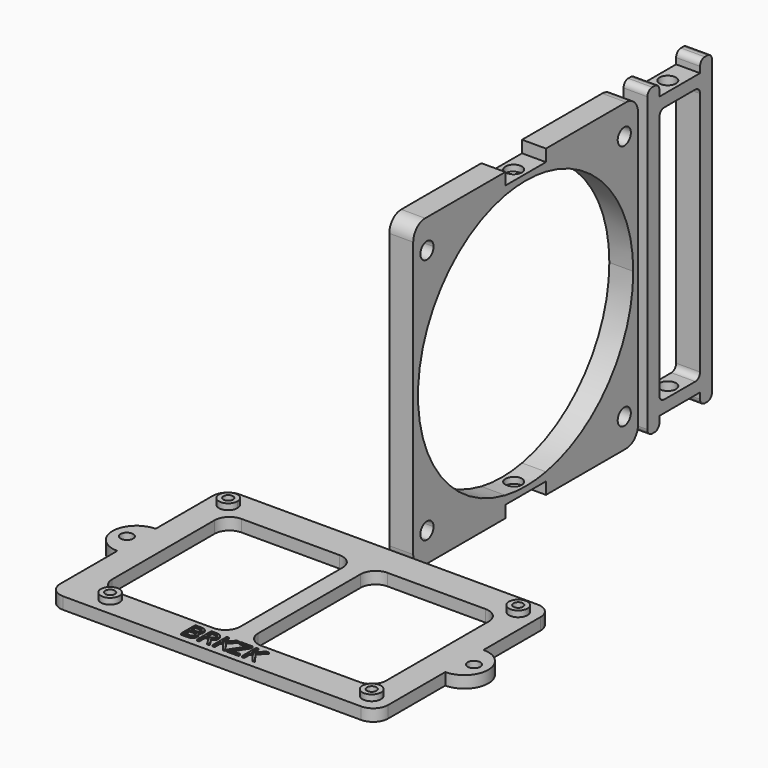
from build123d import *

# Parameters (mm, degrees)
F3_R      = 3.1
F3_W      = 42.85
F3_H      = 52.8
F3_R_2    = 2.1
F3_R_3    = 1.6
F3_W_2    = 0.69140625
F3_H_2    = 0.75
F4_DEPTH  = 4
F5_DEPTH  = 2
F6_DEPTH  = 0.4
F7_R      = 5
F8_R      = 5
F10_R     = 2.75
F10_W     = 38.5
F10_H     = 4
F11_DEPTH = 8
F13_D     = 5.5
F14_R     = 5
F15_W     = 17
F15_H     = 4
F16_DEPTH = 8
F18_D     = 5.5
F19_R     = 2


# Not quite as in the source:
# - a feature names something its author has since deleted; it is built from what else it names


with BuildPart() as f4:
    # F3 (on Top) → F4 (new body)
    with BuildSketch(Plane.XY):
        Polygon((54.85, 36.9), (-54.85, 36.9), (-54.85, 8), (-54.85, -8), (-54.85, -36.9), (-13.0384114583, -36.9), (54.85, -36.9), (54.85, -8), (54.85, 8), align=None)
        with BuildLine():
            Line((-51.85, -33.9), (-51.85, 33.9))
            Line((-51.85, 33.9), (-48.55, 33.9))
            Line((-48.55, 33.9), (51.85, 33.9))
            Line((51.85, 33.9), (51.85, -33.9))
            Line((51.85, -33.9), (11.9448348007, -33.9))
            Line((11.9448348007, -33.9), (12.498046875, -34.65))
            Line((12.498046875, -34.65), (11.6842447917, -34.65))
            Line((11.6842447917, -34.65), (11.1207294487, -33.9))
            Line((11.1207294487, -33.9), (8.892578125, -33.9))
            Line((8.892578125, -33.9), (8.892578125, -34.65))
            Line((8.892578125, -34.65), (8.201171875, -34.65))
            Line((8.201171875, -34.65), (8.201171875, -33.9))
            Line((8.201171875, -33.9), (3.8844248565, -33.9))
            Line((3.8844248565, -33.9), (3.802734375, -34.0236979167))
            Line((3.802734375, -34.0236979167), (7.0501302083, -34.0236979167))
            Line((7.0501302083, -34.0236979167), (7.0501302083, -34.65))
            Line((7.0501302083, -34.65), (2.9602864583, -34.65))
            Line((2.9602864583, -34.65), (2.9602864583, -34.1083333333))
            Line((2.9602864583, -34.1083333333), (3.0977581137, -33.9))
            Line((3.0977581137, -33.9), (2.0737410507, -33.9))
            Line((2.0737410507, -33.9), (2.626953125, -34.65))
            Line((2.626953125, -34.65), (1.8131510417, -34.65))
            Line((1.8131510417, -34.65), (1.2496356987, -33.9))
            Line((1.2496356987, -33.9), (-0.978515625, -33.9))
            Line((-0.978515625, -33.9), (-0.978515625, -34.65))
            Line((-0.978515625, -34.65), (-1.669921875, -34.65))
            Line((-1.669921875, -34.65), (-1.669921875, -33.9))
            Line((-1.669921875, -33.9), (-3.0829182269, -33.9))
            Line((-3.0829182269, -33.9), (-2.6295572917, -34.65))
            Line((-2.6295572917, -34.65), (-3.447265625, -34.65))
            Line((-3.447265625, -34.65), (-3.8838445724, -33.9))
            Line((-3.8838445724, -33.9), (-6.1295572917, -33.9))
            Line((-6.1295572917, -33.9), (-6.1295572917, -34.65))
            Line((-6.1295572917, -34.65), (-6.8209635417, -34.65))
            Line((-6.8209635417, -34.65), (-6.8209635417, -33.9))
            Line((-6.8209635417, -33.9), (-8.3611343756, -33.9))
            add(Edge.make_bspline(
                [(-8.3611343756, -33.9), (-8.4747116287, -34.0669277583), (-8.6373697917, -34.2020833333)],
                knots=[0.6982573208, 0.6982573208, 0.6982573208, 1, 1, 1], degree=2))
            add(Edge.make_bspline(
                [(-8.6373697917, -34.2020833333), (-9.1764322917, -34.65), (-10.1451822917, -34.65)],
                knots=[0, 0, 0, 1, 1, 1], degree=2))
            Line((-10.1451822917, -34.65), (-12.220703125, -34.65))
            Line((-12.220703125, -34.65), (-12.220703125, -33.9))
            Line((-12.220703125, -33.9), (-51.85, -33.9))
        make_face(mode=Mode.SUBTRACT)
        with BuildLine():
            Line((-48.55, 33.9), (-51.85, 33.9))
            Line((-51.85, 33.9), (-51.85, -33.9))
            Line((-51.85, -33.9), (-12.220703125, -33.9))
            Line((-12.220703125, -33.9), (-12.220703125, -28.70078125))
            Line((-12.220703125, -28.70078125), (-10.5397135417, -28.70078125))
            add(Edge.make_bspline(
                [(-10.5397135417, -28.70078125), (-9.3561197917, -28.70078125), (-8.8268229167, -29.0549479167)],
                knots=[0, 0, 0, 1, 1, 1], degree=2))
            add(Edge.make_bspline(
                [(-8.8268229167, -29.0549479167), (-8.2975260417, -29.4091145833), (-8.2975260417, -30.1734375)],
                knots=[0, 0, 0, 1, 1, 1], degree=2))
            add(Edge.make_bspline(
                [(-8.2975260417, -30.1734375), (-8.2975260417, -30.7033854167), (-8.5924479167, -31.0471354167)],
                knots=[0, 0, 0, 1, 1, 1], degree=2))
            add(Edge.make_bspline(
                [(-8.5924479167, -31.0471354167), (-8.8873697917, -31.3908854167), (-9.4537760417, -31.4924479167)],
                knots=[0, 0, 0, 1, 1, 1], degree=2))
            Line((-9.4537760417, -31.4924479167), (-9.4537760417, -31.5328125))
            add(Edge.make_bspline(
                [(-9.4537760417, -31.5328125), (-8.0983072917, -31.7645833333), (-8.0983072917, -32.9572916667)],
                knots=[0, 0, 0, 1, 1, 1], degree=2))
            add(Edge.make_bspline(
                [(-8.0983072917, -32.9572916667), (-8.0983072917, -33.5137154692), (-8.3611343756, -33.9)],
                knots=[0, 0, 0, 0.6982573208, 0.6982573208, 0.6982573208], degree=2))
            Line((-8.3611343756, -33.9), (-6.8209635417, -33.9))
            Line((-6.8209635417, -33.9), (-6.8209635417, -28.70078125))
            Line((-6.8209635417, -28.70078125), (-5.189453125, -28.70078125))
            add(Edge.make_bspline(
                [(-5.189453125, -28.70078125), (-4.0944010417, -28.70078125), (-3.5716145833, -29.1200520833)],
                knots=[0, 0, 0, 1, 1, 1], degree=2))
            add(Edge.make_bspline(
                [(-3.5716145833, -29.1200520833), (-3.048828125, -29.5393229167), (-3.048828125, -30.3817708333)],
                knots=[0, 0, 0, 1, 1, 1], degree=2))
            add(Edge.make_bspline(
                [(-3.048828125, -30.3817708333), (-3.048828125, -31.5614583333), (-4.2454427083, -31.9768229167)],
                knots=[0, 0, 0, 1, 1, 1], degree=2))
            Line((-4.2454427083, -31.9768229167), (-3.0829182269, -33.9))
            Line((-3.0829182269, -33.9), (-1.669921875, -33.9))
            Line((-1.669921875, -33.9), (-1.669921875, -28.70078125))
            Line((-1.669921875, -28.70078125), (-0.978515625, -28.70078125))
            Line((-0.978515625, -28.70078125), (-0.978515625, -31.6513020833))
            Line((-0.978515625, -31.6513020833), (1.7194010417, -28.70078125))
            Line((1.7194010417, -28.70078125), (2.537109375, -28.70078125))
            Line((2.537109375, -28.70078125), (0.1451822917, -31.2854166667))
            Line((0.1451822917, -31.2854166667), (2.0737410507, -33.9))
            Line((2.0737410507, -33.9), (3.0977581137, -33.9))
            Line((3.0977581137, -33.9), (6.1178385417, -29.3231770833))
            Line((6.1178385417, -29.3231770833), (3.0579427083, -29.3231770833))
            Line((3.0579427083, -29.3231770833), (3.0579427083, -28.70078125))
            Line((3.0579427083, -28.70078125), (6.9602864583, -28.70078125))
            Line((6.9602864583, -28.70078125), (6.9602864583, -29.2424479167))
            Line((6.9602864583, -29.2424479167), (3.8844248565, -33.9))
            Line((3.8844248565, -33.9), (8.201171875, -33.9))
            Line((8.201171875, -33.9), (8.201171875, -28.70078125))
            Line((8.201171875, -28.70078125), (8.892578125, -28.70078125))
            Line((8.892578125, -28.70078125), (8.892578125, -31.6513020833))
            Line((8.892578125, -31.6513020833), (11.5904947917, -28.70078125))
            Line((11.5904947917, -28.70078125), (12.408203125, -28.70078125))
            Line((12.408203125, -28.70078125), (10.0162760417, -31.2854166667))
            Line((10.0162760417, -31.2854166667), (11.9448348007, -33.9))
            Line((11.9448348007, -33.9), (51.85, -33.9))
            Line((51.85, -33.9), (51.85, 33.9))
            Line((51.85, 33.9), (-48.55, 33.9))
        make_face()
        with Locations((-39.25, -30.5)):
            Circle(F3_R, mode=Mode.SUBTRACT)
        with Locations((48.25, -30.5)):
            Circle(F3_R, mode=Mode.SUBTRACT)
        Polygon((-45.85, -26.4), (-45.85, 26.4), (-3, 26.4), (-3, -26.4), (-13.0384114583, -26.4), align=None, mode=Mode.SUBTRACT)
        with BuildLine():
            ThreePointArc((-45.45, 30.5), (-50.7420310217, 28.3079689783), (-48.55, 33.6))
            ThreePointArc((-48.55, 33.6), (-46.3579689783, 32.6920310217), (-45.45, 30.5))
        make_face(mode=Mode.SUBTRACT)
        with Locations((24.425, 0)):
            Rectangle(F3_W, F3_H, mode=Mode.SUBTRACT)
        with Locations((48.45, 30.5)):
            Circle(F3_R, mode=Mode.SUBTRACT)
        with BuildLine():
            ThreePointArc((54.85, -8), (62.85, 0), (54.85, 8))
            Line((54.85, 8), (54.85, -8))
        make_face()
        with Locations((58.05, 0)):
            Circle(F3_R_2, mode=Mode.SUBTRACT)
        with BuildLine():
            Line((-54.85, -8), (-54.85, 8))
            ThreePointArc((-54.85, 8), (-62.85, 0), (-54.85, -8))
        make_face()
        with Locations((-58.05, 0)):
            Circle(F3_R_2, mode=Mode.SUBTRACT)
        with BuildLine():
            ThreePointArc((-45.45, 30.5), (-46.3579689783, 32.6920310217), (-48.55, 33.6))
            ThreePointArc((-48.55, 33.6), (-50.7420310217, 28.3079689783), (-45.45, 30.5))
        make_face()
        with BuildLine():
            ThreePointArc((-46.95, 30.5), (-49.6813708499, 29.3686291501), (-48.55, 32.1))
            ThreePointArc((-48.55, 32.1), (-47.4186291501, 31.6313708499), (-46.95, 30.5))
        make_face(mode=Mode.SUBTRACT)
        with Locations((-39.25, -30.5)):
            Circle(F3_R)
        with Locations((-39.25, -30.5)):
            Circle(F3_R_3, mode=Mode.SUBTRACT)
        with Locations((48.25, -30.5)):
            Circle(F3_R)
        with Locations((48.25, -30.5)):
            Circle(F3_R_3, mode=Mode.SUBTRACT)
        with Locations((48.45, 30.5)):
            Circle(F3_R)
        with Locations((48.45, 30.5)):
            Circle(F3_R_3, mode=Mode.SUBTRACT)
        with BuildLine():
            Line((-6.8209635417, -28.70078125), (-6.8209635417, -33.9))
            Line((-6.8209635417, -33.9), (-6.1295572917, -33.9))
            Line((-6.1295572917, -33.9), (-6.1295572917, -32.1760416667))
            Line((-6.1295572917, -32.1760416667), (-4.8873697917, -32.1760416667))
            Line((-4.8873697917, -32.1760416667), (-3.8838445724, -33.9))
            Line((-3.8838445724, -33.9), (-3.0829182269, -33.9))
            Line((-3.0829182269, -33.9), (-4.2454427083, -31.9768229167))
            add(Edge.make_bspline(
                [(-3.048828125, -30.3817708333), (-3.048828125, -31.5614583333), (-4.2454427083, -31.9768229167)],
                knots=[0, 0, 0, 1, 1, 1], degree=2))
            add(Edge.make_bspline(
                [(-3.5716145833, -29.1200520833), (-3.048828125, -29.5393229167), (-3.048828125, -30.3817708333)],
                knots=[0, 0, 0, 1, 1, 1], degree=2))
            add(Edge.make_bspline(
                [(-5.189453125, -28.70078125), (-4.0944010417, -28.70078125), (-3.5716145833, -29.1200520833)],
                knots=[0, 0, 0, 1, 1, 1], degree=2))
            Line((-5.189453125, -28.70078125), (-6.8209635417, -28.70078125))
        make_face()
        with BuildLine():
            Line((-5.1803385417, -31.5822916667), (-6.1295572917, -31.5822916667))
            Line((-6.1295572917, -31.5822916667), (-6.1295572917, -29.3075520833))
            Line((-6.1295572917, -29.3075520833), (-5.2298177083, -29.3075520833))
            add(Edge.make_bspline(
                [(-4.1126302083, -29.56796875), (-4.4602864583, -29.3075520833), (-5.2298177083, -29.3075520833)],
                knots=[0, 0, 0, 1, 1, 1], degree=2))
            add(Edge.make_bspline(
                [(-3.7649739583, -30.4182291667), (-3.7649739583, -29.8283854167), (-4.1126302083, -29.56796875)],
                knots=[0, 0, 0, 1, 1, 1], degree=2))
            add(Edge.make_bspline(
                [(-4.1067708333, -31.2912760417), (-3.7649739583, -31.0002604167), (-3.7649739583, -30.4182291667)],
                knots=[0, 0, 0, 1, 1, 1], degree=2))
            add(Edge.make_bspline(
                [(-5.1803385417, -31.5822916667), (-4.4485677083, -31.5822916667), (-4.1067708333, -31.2912760417)],
                knots=[0, 0, 0, 1, 1, 1], degree=2))
        make_face(mode=Mode.SUBTRACT)
        with BuildLine():
            Line((-12.220703125, -28.70078125), (-12.220703125, -33.9))
            Line((-12.220703125, -33.9), (-11.529296875, -33.9))
            Line((-11.529296875, -33.9), (-11.529296875, -31.83359375))
            Line((-11.529296875, -31.83359375), (-10.3444010417, -31.83359375))
            add(Edge.make_bspline(
                [(-9.2115885417, -32.0940104167), (-9.583984375, -31.83359375), (-10.3444010417, -31.83359375)],
                knots=[0, 0, 0, 1, 1, 1], degree=2))
            add(Edge.make_bspline(
                [(-8.8391927083, -32.9078125), (-8.8391927083, -32.3544270833), (-9.2115885417, -32.0940104167)],
                knots=[0, 0, 0, 1, 1, 1], degree=2))
            add(Edge.make_bspline(
                [(-9.203125, -33.7815104167), (-8.8391927083, -33.5028645833), (-8.8391927083, -32.9078125)],
                knots=[0, 0, 0, 1, 1, 1], degree=2))
            add(Edge.make_bspline(
                [(-9.4000038836, -33.9), (-9.2911480413, -33.8489055181), (-9.203125, -33.7815104167)],
                knots=[0.7581334679, 0.7581334679, 0.7581334679, 1, 1, 1], degree=2))
            Line((-9.4000038836, -33.9), (-8.3611343756, -33.9))
            add(Edge.make_bspline(
                [(-8.0983072917, -32.9572916667), (-8.0983072917, -33.5137154692), (-8.3611343756, -33.9)],
                knots=[0, 0, 0, 0.6982573208, 0.6982573208, 0.6982573208], degree=2))
            add(Edge.make_bspline(
                [(-9.4537760417, -31.5328125), (-8.0983072917, -31.7645833333), (-8.0983072917, -32.9572916667)],
                knots=[0, 0, 0, 1, 1, 1], degree=2))
            Line((-9.4537760417, -31.5328125), (-9.4537760417, -31.4924479167))
            add(Edge.make_bspline(
                [(-8.5924479167, -31.0471354167), (-8.8873697917, -31.3908854167), (-9.4537760417, -31.4924479167)],
                knots=[0, 0, 0, 1, 1, 1], degree=2))
            add(Edge.make_bspline(
                [(-8.2975260417, -30.1734375), (-8.2975260417, -30.7033854167), (-8.5924479167, -31.0471354167)],
                knots=[0, 0, 0, 1, 1, 1], degree=2))
            add(Edge.make_bspline(
                [(-8.8268229167, -29.0549479167), (-8.2975260417, -29.4091145833), (-8.2975260417, -30.1734375)],
                knots=[0, 0, 0, 1, 1, 1], degree=2))
            add(Edge.make_bspline(
                [(-10.5397135417, -28.70078125), (-9.3561197917, -28.70078125), (-8.8268229167, -29.0549479167)],
                knots=[0, 0, 0, 1, 1, 1], degree=2))
            Line((-10.5397135417, -28.70078125), (-12.220703125, -28.70078125))
        make_face()
        with BuildLine():
            Line((-10.3899739583, -31.24765625), (-11.529296875, -31.24765625))
            Line((-11.529296875, -31.24765625), (-11.529296875, -29.2997395833))
            Line((-11.529296875, -29.2997395833), (-10.5110677083, -29.2997395833))
            add(Edge.make_bspline(
                [(-9.3717447917, -29.52109375), (-9.7298177083, -29.2997395833), (-10.5110677083, -29.2997395833)],
                knots=[0, 0, 0, 1, 1, 1], degree=2))
            add(Edge.make_bspline(
                [(-9.013671875, -30.24375), (-9.013671875, -29.7424479167), (-9.3717447917, -29.52109375)],
                knots=[0, 0, 0, 1, 1, 1], degree=2))
            add(Edge.make_bspline(
                [(-9.3352864583, -31.0178385417), (-9.013671875, -30.7880208333), (-9.013671875, -30.24375)],
                knots=[0, 0, 0, 1, 1, 1], degree=2))
            add(Edge.make_bspline(
                [(-10.3899739583, -31.24765625), (-9.6569010417, -31.24765625), (-9.3352864583, -31.0178385417)],
                knots=[0, 0, 0, 1, 1, 1], degree=2))
        make_face(mode=Mode.SUBTRACT)
        Polygon((11.1207294487, -33.9), (11.9448348007, -33.9), (10.0162760417, -31.2854166667), (12.408203125, -28.70078125), (11.5904947917, -28.70078125), (8.892578125, -31.6513020833), (8.892578125, -28.70078125), (8.201171875, -28.70078125), (8.201171875, -33.9), (8.892578125, -33.9), (8.892578125, -32.31796875), (9.5162760417, -31.7645833333), align=None)
        Polygon((1.2496356987, -33.9), (2.0737410507, -33.9), (0.1451822917, -31.2854166667), (2.537109375, -28.70078125), (1.7194010417, -28.70078125), (-0.978515625, -31.6513020833), (-0.978515625, -28.70078125), (-1.669921875, -28.70078125), (-1.669921875, -33.9), (-0.978515625, -33.9), (-0.978515625, -32.31796875), (-0.3548177083, -31.7645833333), align=None)
        Polygon((3.0977581137, -33.9), (3.8844248565, -33.9), (6.9602864583, -29.2424479167), (6.9602864583, -28.70078125), (3.0579427083, -28.70078125), (3.0579427083, -29.3231770833), (6.1178385417, -29.3231770833), align=None)
        with BuildLine():
            Line((-11.529296875, -31.83359375), (-11.529296875, -33.9))
            Line((-11.529296875, -33.9), (-9.4000038836, -33.9))
            add(Edge.make_bspline(
                [(-9.4000038836, -33.9), (-9.2911480413, -33.8489055181), (-9.203125, -33.7815104167)],
                knots=[0.7581334679, 0.7581334679, 0.7581334679, 1, 1, 1], degree=2))
            add(Edge.make_bspline(
                [(-9.203125, -33.7815104167), (-8.8391927083, -33.5028645833), (-8.8391927083, -32.9078125)],
                knots=[0, 0, 0, 1, 1, 1], degree=2))
            add(Edge.make_bspline(
                [(-8.8391927083, -32.9078125), (-8.8391927083, -32.3544270833), (-9.2115885417, -32.0940104167)],
                knots=[0, 0, 0, 1, 1, 1], degree=2))
            add(Edge.make_bspline(
                [(-9.2115885417, -32.0940104167), (-9.583984375, -31.83359375), (-10.3444010417, -31.83359375)],
                knots=[0, 0, 0, 1, 1, 1], degree=2))
            Line((-10.3444010417, -31.83359375), (-11.529296875, -31.83359375))
        make_face()
        with BuildLine():
            Line((-6.1295572917, -29.3075520833), (-6.1295572917, -31.5822916667))
            Line((-6.1295572917, -31.5822916667), (-5.1803385417, -31.5822916667))
            add(Edge.make_bspline(
                [(-5.1803385417, -31.5822916667), (-4.4485677083, -31.5822916667), (-4.1067708333, -31.2912760417)],
                knots=[0, 0, 0, 1, 1, 1], degree=2))
            add(Edge.make_bspline(
                [(-4.1067708333, -31.2912760417), (-3.7649739583, -31.0002604167), (-3.7649739583, -30.4182291667)],
                knots=[0, 0, 0, 1, 1, 1], degree=2))
            add(Edge.make_bspline(
                [(-3.7649739583, -30.4182291667), (-3.7649739583, -29.8283854167), (-4.1126302083, -29.56796875)],
                knots=[0, 0, 0, 1, 1, 1], degree=2))
            add(Edge.make_bspline(
                [(-4.1126302083, -29.56796875), (-4.4602864583, -29.3075520833), (-5.2298177083, -29.3075520833)],
                knots=[0, 0, 0, 1, 1, 1], degree=2))
            Line((-5.2298177083, -29.3075520833), (-6.1295572917, -29.3075520833))
        make_face()
        with BuildLine():
            Line((-11.529296875, -29.2997395833), (-11.529296875, -31.24765625))
            Line((-11.529296875, -31.24765625), (-10.3899739583, -31.24765625))
            add(Edge.make_bspline(
                [(-10.3899739583, -31.24765625), (-9.6569010417, -31.24765625), (-9.3352864583, -31.0178385417)],
                knots=[0, 0, 0, 1, 1, 1], degree=2))
            add(Edge.make_bspline(
                [(-9.3352864583, -31.0178385417), (-9.013671875, -30.7880208333), (-9.013671875, -30.24375)],
                knots=[0, 0, 0, 1, 1, 1], degree=2))
            add(Edge.make_bspline(
                [(-9.013671875, -30.24375), (-9.013671875, -29.7424479167), (-9.3717447917, -29.52109375)],
                knots=[0, 0, 0, 1, 1, 1], degree=2))
            add(Edge.make_bspline(
                [(-9.3717447917, -29.52109375), (-9.7298177083, -29.2997395833), (-10.5110677083, -29.2997395833)],
                knots=[0, 0, 0, 1, 1, 1], degree=2))
            Line((-10.5110677083, -29.2997395833), (-11.529296875, -29.2997395833))
        make_face()
        Polygon((-6.1295572917, -32.1760416667), (-6.1295572917, -33.9), (-3.8838445724, -33.9), (-4.8873697917, -32.1760416667), align=None)
        Polygon((-0.978515625, -33.9), (1.2496356987, -33.9), (-0.3548177083, -31.7645833333), (-0.978515625, -32.31796875), align=None)
        Polygon((8.892578125, -33.9), (11.1207294487, -33.9), (9.5162760417, -31.7645833333), (8.892578125, -32.31796875), align=None)
        Polygon((3.802734375, -34.0236979167), (3.8844248565, -33.9), (3.0977581137, -33.9), (2.9602864583, -34.1083333333), (2.9602864583, -34.65), (7.0501302083, -34.65), (7.0501302083, -34.0236979167), align=None)
        with BuildLine():
            Line((-11.529296875, -33.9), (-12.220703125, -33.9))
            Line((-12.220703125, -33.9), (-12.220703125, -34.65))
            Line((-12.220703125, -34.65), (-10.1451822917, -34.65))
            add(Edge.make_bspline(
                [(-8.6373697917, -34.2020833333), (-9.1764322917, -34.65), (-10.1451822917, -34.65)],
                knots=[0, 0, 0, 1, 1, 1], degree=2))
            add(Edge.make_bspline(
                [(-8.3611343756, -33.9), (-8.4747116287, -34.0669277583), (-8.6373697917, -34.2020833333)],
                knots=[0.6982573208, 0.6982573208, 0.6982573208, 1, 1, 1], degree=2))
            Line((-8.3611343756, -33.9), (-9.4000038836, -33.9))
            add(Edge.make_bspline(
                [(-10.287109375, -34.06015625), (-9.741213792, -34.06015625), (-9.4000038836, -33.9)],
                knots=[0, 0, 0, 0.7581334679, 0.7581334679, 0.7581334679], degree=2))
            Line((-10.287109375, -34.06015625), (-11.529296875, -34.06015625))
            Line((-11.529296875, -34.06015625), (-11.529296875, -33.9))
        make_face()
        Polygon((2.626953125, -34.65), (2.0737410507, -33.9), (1.2496356987, -33.9), (1.8131510417, -34.65), align=None)
        Polygon((12.498046875, -34.65), (11.9448348007, -33.9), (11.1207294487, -33.9), (11.6842447917, -34.65), align=None)
        Polygon((-3.0829182269, -33.9), (-3.8838445724, -33.9), (-3.447265625, -34.65), (-2.6295572917, -34.65), align=None)
        with Locations((-6.4752604167, -34.275)):
            Rectangle(F3_W_2, F3_H_2)
        with Locations((-1.32421875, -34.275)):
            Rectangle(F3_W_2, F3_H_2)
        with Locations((8.546875, -34.275)):
            Rectangle(F3_W_2, F3_H_2)
        with BuildLine():
            Line((-9.4000038836, -33.9), (-11.529296875, -33.9))
            Line((-11.529296875, -33.9), (-11.529296875, -34.06015625))
            Line((-11.529296875, -34.06015625), (-10.287109375, -34.06015625))
            add(Edge.make_bspline(
                [(-10.287109375, -34.06015625), (-9.741213792, -34.06015625), (-9.4000038836, -33.9)],
                knots=[0, 0, 0, 0.7581334679, 0.7581334679, 0.7581334679], degree=2))
        make_face()
    extrude(amount=-F4_DEPTH)

    # F3 (on Top) → F5 (join)
    with BuildSketch(Plane.XY):
        with BuildLine():
            ThreePointArc((-45.45, 30.5), (-46.3579689783, 32.6920310217), (-48.55, 33.6))
            ThreePointArc((-48.55, 33.6), (-50.7420310217, 28.3079689783), (-45.45, 30.5))
        make_face()
        with BuildLine():
            ThreePointArc((-46.95, 30.5), (-49.6813708499, 29.3686291501), (-48.55, 32.1))
            ThreePointArc((-48.55, 32.1), (-47.4186291501, 31.6313708499), (-46.95, 30.5))
        make_face(mode=Mode.SUBTRACT)
        with Locations((-39.25, -30.5)):
            Circle(F3_R)
        with Locations((-39.25, -30.5)):
            Circle(F3_R_3, mode=Mode.SUBTRACT)
        with Locations((48.25, -30.5)):
            Circle(F3_R)
        with Locations((48.25, -30.5)):
            Circle(F3_R_3, mode=Mode.SUBTRACT)
        with Locations((48.45, 30.5)):
            Circle(F3_R)
        with Locations((48.45, 30.5)):
            Circle(F3_R_3, mode=Mode.SUBTRACT)
    extrude(amount=F5_DEPTH)

    # F3 (on Top) → F6 (join)
    with BuildSketch(Plane.XY):
        Polygon((11.1207294487, -33.9), (11.9448348007, -33.9), (10.0162760417, -31.2854166667), (12.408203125, -28.70078125), (11.5904947917, -28.70078125), (8.892578125, -31.6513020833), (8.892578125, -28.70078125), (8.201171875, -28.70078125), (8.201171875, -33.9), (8.892578125, -33.9), (8.892578125, -32.31796875), (9.5162760417, -31.7645833333), align=None)
        with BuildLine():
            Line((-12.220703125, -28.70078125), (-12.220703125, -33.9))
            Line((-12.220703125, -33.9), (-11.529296875, -33.9))
            Line((-11.529296875, -33.9), (-11.529296875, -31.83359375))
            Line((-11.529296875, -31.83359375), (-10.3444010417, -31.83359375))
            add(Edge.make_bspline(
                [(-9.2115885417, -32.0940104167), (-9.583984375, -31.83359375), (-10.3444010417, -31.83359375)],
                knots=[0, 0, 0, 1, 1, 1], degree=2))
            add(Edge.make_bspline(
                [(-8.8391927083, -32.9078125), (-8.8391927083, -32.3544270833), (-9.2115885417, -32.0940104167)],
                knots=[0, 0, 0, 1, 1, 1], degree=2))
            add(Edge.make_bspline(
                [(-9.203125, -33.7815104167), (-8.8391927083, -33.5028645833), (-8.8391927083, -32.9078125)],
                knots=[0, 0, 0, 1, 1, 1], degree=2))
            add(Edge.make_bspline(
                [(-9.4000038836, -33.9), (-9.2911480413, -33.8489055181), (-9.203125, -33.7815104167)],
                knots=[0.7581334679, 0.7581334679, 0.7581334679, 1, 1, 1], degree=2))
            Line((-9.4000038836, -33.9), (-8.3611343756, -33.9))
            add(Edge.make_bspline(
                [(-8.0983072917, -32.9572916667), (-8.0983072917, -33.5137154692), (-8.3611343756, -33.9)],
                knots=[0, 0, 0, 0.6982573208, 0.6982573208, 0.6982573208], degree=2))
            add(Edge.make_bspline(
                [(-9.4537760417, -31.5328125), (-8.0983072917, -31.7645833333), (-8.0983072917, -32.9572916667)],
                knots=[0, 0, 0, 1, 1, 1], degree=2))
            Line((-9.4537760417, -31.5328125), (-9.4537760417, -31.4924479167))
            add(Edge.make_bspline(
                [(-8.5924479167, -31.0471354167), (-8.8873697917, -31.3908854167), (-9.4537760417, -31.4924479167)],
                knots=[0, 0, 0, 1, 1, 1], degree=2))
            add(Edge.make_bspline(
                [(-8.2975260417, -30.1734375), (-8.2975260417, -30.7033854167), (-8.5924479167, -31.0471354167)],
                knots=[0, 0, 0, 1, 1, 1], degree=2))
            add(Edge.make_bspline(
                [(-8.8268229167, -29.0549479167), (-8.2975260417, -29.4091145833), (-8.2975260417, -30.1734375)],
                knots=[0, 0, 0, 1, 1, 1], degree=2))
            add(Edge.make_bspline(
                [(-10.5397135417, -28.70078125), (-9.3561197917, -28.70078125), (-8.8268229167, -29.0549479167)],
                knots=[0, 0, 0, 1, 1, 1], degree=2))
            Line((-10.5397135417, -28.70078125), (-12.220703125, -28.70078125))
        make_face()
        with BuildLine():
            Line((-10.3899739583, -31.24765625), (-11.529296875, -31.24765625))
            Line((-11.529296875, -31.24765625), (-11.529296875, -29.2997395833))
            Line((-11.529296875, -29.2997395833), (-10.5110677083, -29.2997395833))
            add(Edge.make_bspline(
                [(-9.3717447917, -29.52109375), (-9.7298177083, -29.2997395833), (-10.5110677083, -29.2997395833)],
                knots=[0, 0, 0, 1, 1, 1], degree=2))
            add(Edge.make_bspline(
                [(-9.013671875, -30.24375), (-9.013671875, -29.7424479167), (-9.3717447917, -29.52109375)],
                knots=[0, 0, 0, 1, 1, 1], degree=2))
            add(Edge.make_bspline(
                [(-9.3352864583, -31.0178385417), (-9.013671875, -30.7880208333), (-9.013671875, -30.24375)],
                knots=[0, 0, 0, 1, 1, 1], degree=2))
            add(Edge.make_bspline(
                [(-10.3899739583, -31.24765625), (-9.6569010417, -31.24765625), (-9.3352864583, -31.0178385417)],
                knots=[0, 0, 0, 1, 1, 1], degree=2))
        make_face(mode=Mode.SUBTRACT)
        with BuildLine():
            Line((-11.529296875, -33.9), (-12.220703125, -33.9))
            Line((-12.220703125, -33.9), (-12.220703125, -34.65))
            Line((-12.220703125, -34.65), (-10.1451822917, -34.65))
            add(Edge.make_bspline(
                [(-8.6373697917, -34.2020833333), (-9.1764322917, -34.65), (-10.1451822917, -34.65)],
                knots=[0, 0, 0, 1, 1, 1], degree=2))
            add(Edge.make_bspline(
                [(-8.3611343756, -33.9), (-8.4747116287, -34.0669277583), (-8.6373697917, -34.2020833333)],
                knots=[0.6982573208, 0.6982573208, 0.6982573208, 1, 1, 1], degree=2))
            Line((-8.3611343756, -33.9), (-9.4000038836, -33.9))
            add(Edge.make_bspline(
                [(-10.287109375, -34.06015625), (-9.741213792, -34.06015625), (-9.4000038836, -33.9)],
                knots=[0, 0, 0, 0.7581334679, 0.7581334679, 0.7581334679], degree=2))
            Line((-10.287109375, -34.06015625), (-11.529296875, -34.06015625))
            Line((-11.529296875, -34.06015625), (-11.529296875, -33.9))
        make_face()
        with BuildLine():
            Line((-6.8209635417, -28.70078125), (-6.8209635417, -33.9))
            Line((-6.8209635417, -33.9), (-6.1295572917, -33.9))
            Line((-6.1295572917, -33.9), (-6.1295572917, -32.1760416667))
            Line((-6.1295572917, -32.1760416667), (-4.8873697917, -32.1760416667))
            Line((-4.8873697917, -32.1760416667), (-3.8838445724, -33.9))
            Line((-3.8838445724, -33.9), (-3.0829182269, -33.9))
            Line((-3.0829182269, -33.9), (-4.2454427083, -31.9768229167))
            add(Edge.make_bspline(
                [(-3.048828125, -30.3817708333), (-3.048828125, -31.5614583333), (-4.2454427083, -31.9768229167)],
                knots=[0, 0, 0, 1, 1, 1], degree=2))
            add(Edge.make_bspline(
                [(-3.5716145833, -29.1200520833), (-3.048828125, -29.5393229167), (-3.048828125, -30.3817708333)],
                knots=[0, 0, 0, 1, 1, 1], degree=2))
            add(Edge.make_bspline(
                [(-5.189453125, -28.70078125), (-4.0944010417, -28.70078125), (-3.5716145833, -29.1200520833)],
                knots=[0, 0, 0, 1, 1, 1], degree=2))
            Line((-5.189453125, -28.70078125), (-6.8209635417, -28.70078125))
        make_face()
        with BuildLine():
            Line((-5.1803385417, -31.5822916667), (-6.1295572917, -31.5822916667))
            Line((-6.1295572917, -31.5822916667), (-6.1295572917, -29.3075520833))
            Line((-6.1295572917, -29.3075520833), (-5.2298177083, -29.3075520833))
            add(Edge.make_bspline(
                [(-4.1126302083, -29.56796875), (-4.4602864583, -29.3075520833), (-5.2298177083, -29.3075520833)],
                knots=[0, 0, 0, 1, 1, 1], degree=2))
            add(Edge.make_bspline(
                [(-3.7649739583, -30.4182291667), (-3.7649739583, -29.8283854167), (-4.1126302083, -29.56796875)],
                knots=[0, 0, 0, 1, 1, 1], degree=2))
            add(Edge.make_bspline(
                [(-4.1067708333, -31.2912760417), (-3.7649739583, -31.0002604167), (-3.7649739583, -30.4182291667)],
                knots=[0, 0, 0, 1, 1, 1], degree=2))
            add(Edge.make_bspline(
                [(-5.1803385417, -31.5822916667), (-4.4485677083, -31.5822916667), (-4.1067708333, -31.2912760417)],
                knots=[0, 0, 0, 1, 1, 1], degree=2))
        make_face(mode=Mode.SUBTRACT)
        with Locations((-6.4752604167, -34.275)):
            Rectangle(F3_W_2, F3_H_2)
        Polygon((-3.0829182269, -33.9), (-3.8838445724, -33.9), (-3.447265625, -34.65), (-2.6295572917, -34.65), align=None)
        Polygon((1.2496356987, -33.9), (2.0737410507, -33.9), (0.1451822917, -31.2854166667), (2.537109375, -28.70078125), (1.7194010417, -28.70078125), (-0.978515625, -31.6513020833), (-0.978515625, -28.70078125), (-1.669921875, -28.70078125), (-1.669921875, -33.9), (-0.978515625, -33.9), (-0.978515625, -32.31796875), (-0.3548177083, -31.7645833333), align=None)
        with Locations((-1.32421875, -34.275)):
            Rectangle(F3_W_2, F3_H_2)
        Polygon((2.626953125, -34.65), (2.0737410507, -33.9), (1.2496356987, -33.9), (1.8131510417, -34.65), align=None)
        Polygon((3.0977581137, -33.9), (3.8844248565, -33.9), (6.9602864583, -29.2424479167), (6.9602864583, -28.70078125), (3.0579427083, -28.70078125), (3.0579427083, -29.3231770833), (6.1178385417, -29.3231770833), align=None)
        Polygon((3.802734375, -34.0236979167), (3.8844248565, -33.9), (3.0977581137, -33.9), (2.9602864583, -34.1083333333), (2.9602864583, -34.65), (7.0501302083, -34.65), (7.0501302083, -34.0236979167), align=None)
        with Locations((8.546875, -34.275)):
            Rectangle(F3_W_2, F3_H_2)
        Polygon((12.498046875, -34.65), (11.9448348007, -33.9), (11.1207294487, -33.9), (11.6842447917, -34.65), align=None)
    extrude(amount=F6_DEPTH)

    # F7
    f7_edges = [f4.edges().sort_by_distance(p)[0] for p in [
        (-54.85, -36.9, -2),
        (-54.85, 36.9, -2),
        (54.85, -36.9, -2),
        (54.85, 36.9, -2),
    ]]
    fillet(f7_edges, radius=F7_R)

    # F8
    f8_edges = [f4.edges().sort_by_distance(p)[0] for p in [
        (-45.85, 26.4, -2),
        (45.85, 26.4, -2),
        (-45.85, -26.4, -2),
        (45.85, -26.4, -2),
        (3, 26.4, -2),
        (-3, 26.4, -2),
        (-3, -26.4, -2),
        (3, -26.4, -2),
    ]]
    fillet(f8_edges, radius=F8_R)


with BuildPart() as f11:
    # F10 (on Right) → F11 (new body)
    with BuildSketch(Plane.YZ):
        with BuildLine():
            Line((131.1611504041, 94), (92.6611504041, 94))
            Line((92.6611504041, 94), (92.6611504041, 91.1899309798))
            ThreePointArc((92.6611504041, 91.1899309798), (118.8562509227, 75.6574597618), (129.1611504041, 47))
            ThreePointArc((129.1611504041, 47), (118.8562509227, 18.3425402382), (92.6611504041, 2.8100690202))
            Line((92.6611504041, 2.8100690202), (92.6611504041, 0))
            Line((92.6611504041, 0), (131.1611504041, 0))
            Line((131.1611504041, 0), (131.1611504041, 5.75))
            Line((131.1611504041, 5.75), (131.1611504041, 94))
        make_face()
        with Locations((125.4111504041, 5.75)):
            Circle(F10_R, mode=Mode.SUBTRACT)
        with Locations((125.4111504041, 88.25)):
            Circle(F10_R, mode=Mode.SUBTRACT)
        with BuildLine():
            Line((40.1611504041, 5.75), (37.1611504041, 5.75))
            Line((37.1611504041, 5.75), (37.1611504041, 0))
            Line((37.1611504041, 0), (42.9111504041, 0))
            Line((42.9111504041, 0), (42.9111504041, 3))
            ThreePointArc((42.9111504041, 3), (40.9666067558, 3.8054563517), (40.1611504041, 5.75))
        make_face()
        Polygon((42.9111504041, 0), (37.1611504041, 0), (37.1611504041, -4), (75.6611504041, -4), (75.6611504041, 0), align=None)
        with Locations((111.9111504041, -2)):
            Rectangle(F10_W, F10_H)
        with BuildLine():
            ThreePointArc((92.6611504041, 2.8100690202), (84.1611504041, 2), (75.6611504041, 2.8100690202))
            Line((75.6611504041, 2.8100690202), (75.6611504041, 0))
            Line((75.6611504041, 0), (92.6611504041, 0))
            Line((92.6611504041, 0), (92.6611504041, 2.8100690202))
        make_face()
        with BuildLine():
            Line((92.6611504041, 94), (75.6611504041, 94))
            Line((75.6611504041, 94), (75.6611504041, 91.1899309798))
            ThreePointArc((75.6611504041, 91.1899309798), (84.1611504041, 92), (92.6611504041, 91.1899309798))
            Line((92.6611504041, 91.1899309798), (92.6611504041, 94))
        make_face()
        with Locations((111.9111504041, 96)):
            Rectangle(F10_W, F10_H)
        Polygon((37.1611504041, 98), (37.1611504041, 94), (42.9111504041, 94), (75.6611504041, 94), (75.6611504041, 98), align=None)
        with BuildLine():
            Line((42.9111504041, 94), (37.1611504041, 94))
            Line((37.1611504041, 94), (37.1611504041, 5.75))
            Line((37.1611504041, 5.75), (40.1611504041, 5.75))
            ThreePointArc((40.1611504041, 5.75), (42.9111504041, 8.5), (45.6611504041, 5.75))
            ThreePointArc((45.6611504041, 5.75), (44.8556940523, 3.8054563517), (42.9111504041, 3))
            Line((42.9111504041, 3), (42.9111504041, 0))
            Line((42.9111504041, 0), (75.6611504041, 0))
            Line((75.6611504041, 0), (75.6611504041, 2.8100690202))
            ThreePointArc((75.6611504041, 2.8100690202), (39.1611504041, 47), (75.6611504041, 91.1899309798))
            Line((75.6611504041, 91.1899309798), (75.6611504041, 94))
            Line((75.6611504041, 94), (42.9111504041, 94))
        make_face()
        with BuildLine():
            ThreePointArc((45.6611504041, 88.25), (40.9666067558, 86.3054563517), (42.9111504041, 91))
            ThreePointArc((42.9111504041, 91), (44.8556940523, 90.1945436483), (45.6611504041, 88.25))
        make_face(mode=Mode.SUBTRACT)
    extrude(amount=F11_DEPTH)

    # F13 (through all)
    with Locations(Plane(origin=(0, 0, 0), x_dir=(1, 0, 0), z_dir=(0, 0, -1))):
        with Locations((4, -84.1611504041)):
            Hole(F13_D / 2)

    # F14
    f14_edges = [f11.edges().sort_by_distance(p)[0] for p in [
        (4, 131.16115, 98),
        (4, 37.16115, 98),
        (4, 131.16115, -4),
        (4, 37.16115, -4),
    ]]
    fillet(f14_edges, radius=F14_R)


with BuildPart() as f16:
    # F15 (on Right) → F16 (new body)
    with BuildSketch(Plane.YZ):
        Polygon((157.0976424254, 4), (157.0976424254, 0), (157.0976424254, -4), (162.0976424254, -4), (162.0976424254, 98), (157.0976424254, 98), (157.0976424254, 94), (157.0976424254, 90), align=None)
        with Locations((148.5976424254, 2)):
            Rectangle(F15_W, F15_H)
        Polygon((140.0976424254, -4), (140.0976424254, 0), (140.0976424254, 4), (140.0976424254, 90), (140.0976424254, 94), (140.0976424254, 98), (135.0976424254, 98), (135.0976424254, -4), align=None)
        with Locations((148.5976424254, 92)):
            Rectangle(F15_W, F15_H)
    extrude(amount=F16_DEPTH)

    # F18 (through all)
    with Locations(Plane.XY.offset(94)):
        with Locations((4, 148.5976424254)):
            Hole(F18_D / 2)

    # F19
    f19_edges = [f16.edges().sort_by_distance(p)[0] for p in [
        (4, 135.097642, -4),
        (4, 140.097642, -4),
        (4, 157.097642, -4),
        (4, 162.097642, -4),
        (4, 162.097642, 98),
        (4, 157.097642, 98),
        (4, 140.097642, 98),
        (4, 135.097642, 98),
        (4, 140.097642, 90),
        (4, 157.097642, 90),
        (4, 140.097642, 4),
        (4, 157.097642, 4),
    ]]
    fillet(f19_edges, radius=F19_R)


solid = Compound([f4.part, f11.part, f16.part])
